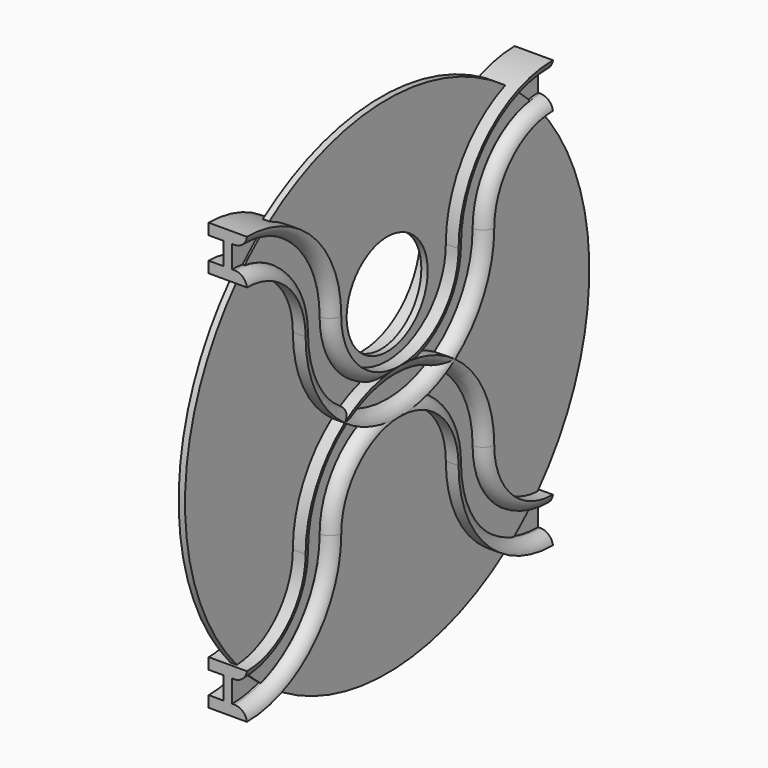
from build123d import *

# Parameters (mm, degrees)
F3_T2_ANGLE = 106.9758894245
F3_T4_ANGLE = 111.4600866309
F4_T2_ANGLE = 111.4600866309
F4_T4_ANGLE = 106.9758894245
F7_R        = 1006.8447254847
F7_R_2      = 201.8351367634
F8_DEPTH    = 25.4


# Not quite as in the source:
# - a fillet or chamfer that OpenCascade refuses, or shapes differently, is made with other operations: its cross-section is extruded or revolved along the edge and cut away or added
# - a feature of the source that left no trace in its solid (it failed there, or was rolled back) is left out


with BuildPart() as f2:
    # F2: sweep along a path in F1
    with BuildLine(Plane.YZ) as f2_path:
        ThreePointArc((0, 0), (269.4076836321, -111.5923163679), (381, -381))
        ThreePointArc((381, -381), (492.5923163679, -650.4076836321), (762, -762))
    # F0 (on Front) → F2 (sweep)
    with BuildSketch(Plane.XZ):
        Polygon((76.2, 88.9), (0, 88.9), (-76.2, 88.9), (-76.2, 44.45), (-17.3748321831, 44.45), (-17.3748321831, 0), (-17.3748321831, -44.45), (-76.2, -44.45), (-76.2, -88.9), (0, -88.9), (76.2, -88.9), (76.2, -44.45), (17.3748321831, -44.45), (17.3748321831, 0), (17.3748321831, 44.45), (76.2, 44.45), align=None)
    sweep(path=f2_path.line)

    # F3: fillet of radius 50.8 on 2 edges, made by hand

    # F3_s1 → F3_t2 (revolve, cut)
    with BuildSketch(Plane(origin=(0, -106.3932922966, -32.4787439795), x_dir=(1, 0, 0), z_dir=(0, -0.9564277039, -0.2919692573))):
        with BuildLine():
            ThreePointArc((76.2, 105.5010448097), (59.3994791747, 73.7510448097), (25.7984375242, 61.0510448097))
            Line((25.7984375242, 61.0510448097), (76.2, 61.0510448097))
            Line((76.2, 61.0510448097), (76.2, 105.5010448097))
        make_face()
    revolve(axis=Axis((76.2, 0, -381), (-1, 0, 0)), revolution_arc=F3_T2_ANGLE, mode=Mode.SUBTRACT)

    # F3_s3 → F3_t4 (revolve, cut)
    with BuildSketch(Plane.XY.offset(-381)):
        with BuildLine():
            ThreePointArc((76.2, 469.9), (59.3994791747, 438.15), (25.7984375242, 425.45))
            Line((25.7984375242, 425.45), (76.2, 425.45))
            Line((76.2, 425.45), (76.2, 469.9))
        make_face()
    revolve(axis=Axis((76.2, 762, -381), (1, 0, 0)), revolution_arc=F3_T4_ANGLE, mode=Mode.SUBTRACT)

    # F4: fillet of radius 50.8 on 2 edges, made by hand

    # F4_s1 → F4_t2 (revolve, cut)
    with BuildSketch(Plane(origin=(0, -129.7264514316, -50.9962444987), x_dir=(1, 0, 0), z_dir=(0, -0.9306726542, -0.3658529906))):
        with BuildLine():
            ThreePointArc((25.7984375242, -18.0362812434), (59.3994791747, -30.7362812434), (76.2, -62.4862812434))
            Line((76.2, -62.4862812434), (76.2, -18.0362812434))
            Line((76.2, -18.0362812434), (25.7984375242, -18.0362812434))
        make_face()
    revolve(axis=Axis((76.2, 0, -381), (-1, 0, 0)), revolution_arc=F4_T2_ANGLE, mode=Mode.SUBTRACT)

    # F4_s3 → F4_t4 (revolve, cut)
    with BuildSketch(Plane.XY.offset(-381)):
        with BuildLine():
            ThreePointArc((25.7984375242, 336.55), (59.3994791747, 323.85), (76.2, 292.1))
            Line((76.2, 292.1), (76.2, 336.55))
            Line((76.2, 336.55), (25.7984375242, 336.55))
        make_face()
    revolve(axis=Axis((76.2, 762, -381), (1, 0, 0)), revolution_arc=F4_T4_ANGLE, mode=Mode.SUBTRACT)

    # F5: F2 across plane


with BuildPart() as f2_1:
    add(f2.part)
    add(f2.part.mirror(Plane.XZ))

    # F6: F2 across plane


with BuildPart() as f2_2:
    add(f2_1.part)
    add(f2_1.part.mirror(Plane.XY))

    # F7 (on Right) → F8 (join)
    with BuildSketch(Plane.YZ):
        Circle(F7_R)
        with Locations((0, 323.4876990318)):
            Circle(F7_R_2, mode=Mode.SUBTRACT)
    extrude(amount=F8_DEPTH)


solid = f2_2.part
